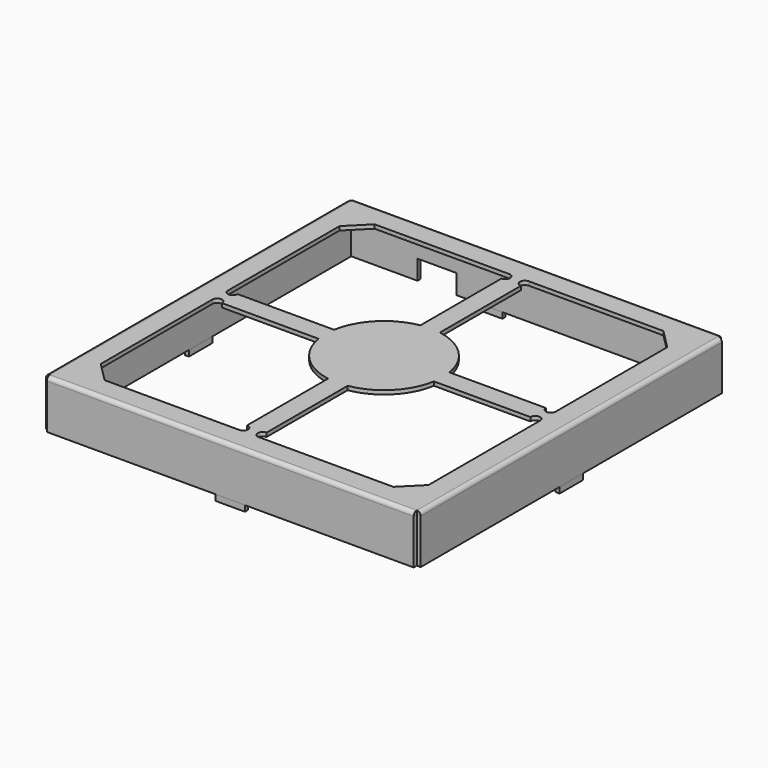
from build123d import *

# Parameters (mm, degrees)
F1_START = 2.3
F0_W     = 8.65
F0_H     = 0.2
F0_W_2   = 1.5
F0_W_3   = 0.2
F0_H_2   = 8.9
F0_H_3   = 1.5
F0_W_4   = 11.05
F0_W_5   = 0.85
F0_W_6   = 2
F0_W_7   = 3.4
F1_DEPTH = 0.2
F2_DEPTH = 2.3
F3_DEPTH = 0.3
F4_DEPTH = 1
F5_R     = 0.1999


# Not quite as in the source:
# - a fillet or chamfer is up to 0.001 mm smaller than in the source, because OpenCascade refuses the exact size
# - ends of sketch curves that miss each other by under 0.0002 mm in the source are joined


with BuildPart() as f1:
    # F0 (on Top) → F1 (new body)
    with BuildSketch(Plane.XY.offset(F1_START)):
        Polygon((-6, 9.65), (-9.4, 9.65), (-9.4, 0.75), (-9.4, -0.75), (-9.4, -9.65), (-0.75, -9.65), (0.75, -9.65), (9.4, -9.65), (9.4, -0.75), (9.4, 0.75), (9.4, 9.65), (-1.65, 9.65), (-3.15, 9.65), (-4, 9.65), align=None)
        with BuildLine():
            Line((-0.5, -8.65), (-7.4, -8.65))
            Line((-7.4, -8.65), (-8.4, -7.65))
            Line((-8.4, -7.65), (-8.4, -0.5))
            ThreePointArc((-8.4, -0.5), (-8.15, -0.25), (-7.9, -0.5))
            Line((-7.9, -0.5), (-2.95804, -0.5))
            ThreePointArc((-2.95804, -0.5), (-2.1213203436, -2.1213203436), (-0.4999999822, -2.9580398946))
            Line((-0.4999999822, -2.9580398946), (-0.5, -8.15))
            ThreePointArc((-0.5, -8.15), (-0.25, -8.4), (-0.5, -8.65))
        make_face(mode=Mode.SUBTRACT)
        with BuildLine():
            Line((8.4, -7.65), (7.4, -8.65))
            Line((7.4, -8.65), (0.5, -8.65))
            ThreePointArc((0.5, -8.65), (0.25, -8.4), (0.5, -8.15))
            Line((0.5, -8.15), (0.5, -2.95804))
            ThreePointArc((0.5, -2.95804), (2.1213203436, -2.1213203436), (2.9580398946, -0.4999999822))
            Line((2.9580398946, -0.4999999822), (7.9, -0.5))
            ThreePointArc((7.9, -0.5), (8.15, -0.25), (8.4, -0.5))
            Line((8.4, -0.5), (8.4, -7.65))
        make_face(mode=Mode.SUBTRACT)
        with BuildLine():
            Line((-8.4, 0.5), (-8.4, 7.65))
            Line((-8.4, 7.65), (-7.4, 8.65))
            Line((-7.4, 8.65), (-0.5, 8.65))
            ThreePointArc((-0.5, 8.65), (-0.25, 8.4), (-0.5, 8.15))
            Line((-0.5, 8.15), (-0.5, 2.95804))
            ThreePointArc((-0.5, 2.95804), (-2.1213203436, 2.1213203436), (-2.9580398946, 0.4999999822))
            Line((-2.9580398946, 0.4999999822), (-7.9, 0.5))
            ThreePointArc((-7.9, 0.5), (-8.15, 0.25), (-8.4, 0.5))
        make_face(mode=Mode.SUBTRACT)
        with BuildLine():
            Line((0.5, 8.65), (7.4, 8.65))
            Line((7.4, 8.65), (8.4, 7.65))
            Line((8.4, 7.65), (8.4, 0.5))
            ThreePointArc((8.4, 0.5), (8.15, 0.25), (7.9, 0.5))
            Line((7.9, 0.5), (2.95804, 0.5))
            ThreePointArc((2.95804, 0.5), (2.1213203436, 2.1213203436), (0.4999999822, 2.9580398946))
            Line((0.4999999822, 2.9580398946), (0.5, 8.15))
            ThreePointArc((0.5, 8.15), (0.25, 8.4), (0.5, 8.65))
        make_face(mode=Mode.SUBTRACT)
        with Locations((-5.075, -9.75)):
            Rectangle(F0_W, F0_H)
        with Locations((0, -9.75)):
            Rectangle(F0_W_2, F0_H)
        with Locations((5.075, -9.75)):
            Rectangle(F0_W, F0_H)
        with Locations((9.5, -5.2)):
            Rectangle(F0_W_3, F0_H_2)
        with Locations((9.5, 0)):
            Rectangle(F0_W_3, F0_H_3)
        with Locations((9.5, 5.2)):
            Rectangle(F0_W_3, F0_H_2)
        with Locations((3.875, 9.75)):
            Rectangle(F0_W_4, F0_H)
        with Locations((-2.4, 9.75)):
            Rectangle(F0_W_2, F0_H)
        with Locations((-3.575, 9.75)):
            Rectangle(F0_W_5, F0_H)
        with Locations((-5, 9.75)):
            Rectangle(F0_W_6, F0_H)
        with Locations((-7.7, 9.75)):
            Rectangle(F0_W_7, F0_H)
        with Locations((-9.5, 5.2)):
            Rectangle(F0_W_3, F0_H_2)
        with Locations((-9.5, 0)):
            Rectangle(F0_W_3, F0_H_3)
        with Locations((-9.5, -5.2)):
            Rectangle(F0_W_3, F0_H_2)
    extrude(amount=F1_DEPTH)

    # F5 (radius 0.2 in the source; OpenCascade refuses exactly that, so slightly less here)
    f5_edges = [f1.edges().sort_by_distance(p)[0] for p in [
        (0, -9.85, 2.5),
        (9.6, 0, 2.5),
        (0, 9.85, 2.5),
        (-9.6, 0, 2.5),
    ]]
    fillet(f5_edges, radius=F5_R)


with BuildPart() as f2:
    # F0 (on Top) → F2 (new body)
    with BuildSketch(Plane.XY):
        with Locations((-5.075, -9.75)):
            Rectangle(F0_W, F0_H)
        with Locations((0, -9.75)):
            Rectangle(F0_W_2, F0_H)
        with Locations((5.075, -9.75)):
            Rectangle(F0_W, F0_H)
    extrude(amount=F2_DEPTH)


with BuildPart() as f2b:
    # F0 (on Top) → F2, piece 2 (new body)
    with BuildSketch(Plane.XY):
        with Locations((9.5, -5.2)):
            Rectangle(F0_W_3, F0_H_2)
        with Locations((9.5, 0)):
            Rectangle(F0_W_3, F0_H_3)
        with Locations((9.5, 5.2)):
            Rectangle(F0_W_3, F0_H_2)
    extrude(amount=F2_DEPTH)


with BuildPart() as f2c:
    # F0 (on Top) → F2, piece 3 (new body)
    with BuildSketch(Plane.XY):
        with Locations((3.875, 9.75)):
            Rectangle(F0_W_4, F0_H)
        with Locations((-2.4, 9.75)):
            Rectangle(F0_W_2, F0_H)
        with Locations((-3.575, 9.75)):
            Rectangle(F0_W_5, F0_H)
        with Locations((-5, 9.75)):
            Rectangle(F0_W_6, F0_H)
        with Locations((-7.7, 9.75)):
            Rectangle(F0_W_7, F0_H)
    extrude(amount=F2_DEPTH)

    # F0 (on Top) → F4 (cut)
    with BuildSketch(Plane.XY):
        with Locations((-5, 9.75)):
            Rectangle(F0_W_6, F0_H)
    extrude(amount=F4_DEPTH, mode=Mode.SUBTRACT)


with BuildPart() as f2d:
    # F0 (on Top) → F2, piece 4 (new body)
    with BuildSketch(Plane.XY):
        with Locations((-9.5, 5.2)):
            Rectangle(F0_W_3, F0_H_2)
        with Locations((-9.5, 0)):
            Rectangle(F0_W_3, F0_H_3)
        with Locations((-9.5, -5.2)):
            Rectangle(F0_W_3, F0_H_2)
    extrude(amount=F2_DEPTH)


with BuildPart() as f3:
    # F0 (on Top) → F3 (new body)
    with BuildSketch(Plane.XY):
        with Locations((9.5, 0)):
            Rectangle(F0_W_3, F0_H_3)
    extrude(amount=-F3_DEPTH)


with BuildPart() as f3b:
    # F0 (on Top) → F3, piece 2 (new body)
    with BuildSketch(Plane.XY):
        with Locations((0, -9.75)):
            Rectangle(F0_W_2, F0_H)
    extrude(amount=-F3_DEPTH)


with BuildPart() as f3c:
    # F0 (on Top) → F3, piece 3 (new body)
    with BuildSketch(Plane.XY):
        with Locations((-9.5, 0)):
            Rectangle(F0_W_3, F0_H_3)
    extrude(amount=-F3_DEPTH)


with BuildPart() as f3d:
    # F0 (on Top) → F3, piece 4 (new body)
    with BuildSketch(Plane.XY):
        with Locations((-2.4, 9.75)):
            Rectangle(F0_W_2, F0_H)
    extrude(amount=-F3_DEPTH)


solid = Compound([f1.part, f2.part, f2b.part, f2c.part, f2d.part, f3.part, f3b.part, f3c.part, f3d.part])
